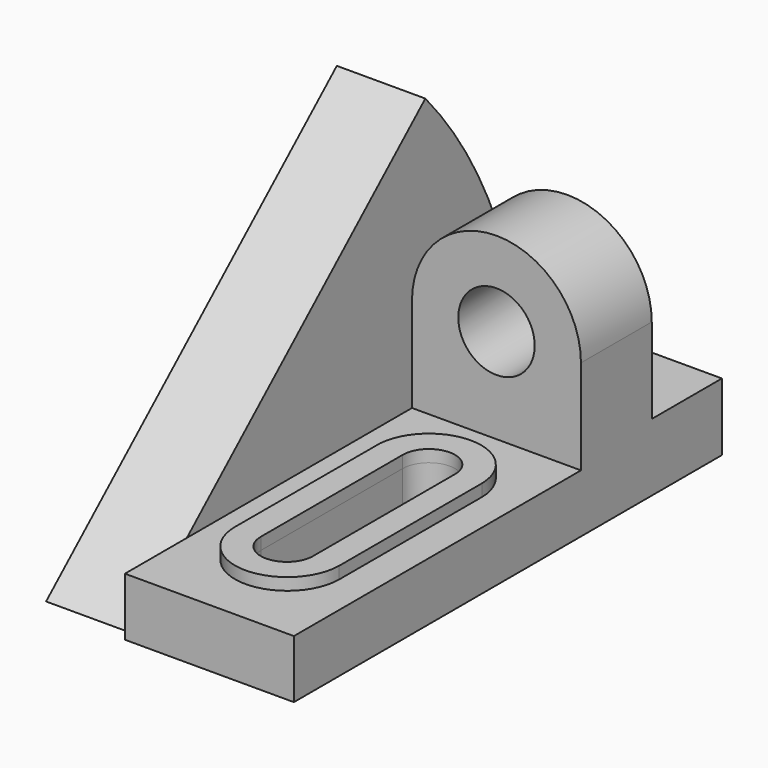
from build123d import *
from build123d import SkipClean  # not in build123d's __all__

# Parameters (mm, degrees)
F0_W          = 42
F0_H          = 16
F0_R          = 9.5
F1_DEPTH      = 133
F2_W          = 35.961864282
F2_H          = 49.2198635868
F3_DEPTH      = 23.6373633247
F3_DEPTH_BACK = 25
F4_W          = 102.4302720154
F4_H          = 59.7613004169
F5_DEPTH      = 25
F5_DEPTH_BACK = 25
F7_DEPTH      = 22
F9_DEPTH      = 25
F10_DEPTH     = 3


with BuildPart() as f1:
    # F0 (on Front) → F1 (new body)
    with BuildSketch(Plane.XZ):
        with Locations((-2.6363633247, 8)):
            Rectangle(F0_W, F0_H)
        with BuildLine():
            Line((-23.6363633247, 38), (-23.6363633247, 16))
            Line((-23.6363633247, 16), (18.3636366753, 16))
            Line((18.3636366753, 16), (18.3636366753, 38))
            ThreePointArc((18.3636366753, 38), (-2.6363633247, 59), (-23.6363633247, 38))
        make_face()
        with Locations((-2.6363633247, 38)):
            Circle(F0_R, mode=Mode.SUBTRACT)
    extrude(amount=F1_DEPTH)

    # F2 (on Right) → F3 (cut, two sides)
    with BuildSketch(Plane.YZ) as f3_sk:
        with Locations((-3.8203388158, 41.385004092)):
            Rectangle(F2_W, F2_H)
    extrude(amount=-F3_DEPTH, mode=Mode.SUBTRACT)
    extrude(f3_sk.sketch, amount=F3_DEPTH_BACK, mode=Mode.SUBTRACT)

    # F4 (on Right) → F5 (cut, two sides)
    with BuildSketch(Plane.YZ) as f5_sk:
        with Locations((-95.0164069645, 44.3436447531)):
            Rectangle(F4_W, F4_H)
    extrude(amount=-F5_DEPTH, mode=Mode.SUBTRACT)
    extrude(f5_sk.sketch, amount=F5_DEPTH_BACK, mode=Mode.SUBTRACT)

    # F6 (on face) → F7 (join)
    with BuildSketch(Plane(origin=(-23.6363633247, 0, 0), x_dir=(0, -1, 0), z_dir=(-1, 0, 0))):
        with BuildLine():
            Line((9, 0), (130, 0))
            Line((130, 0), (39.6567079743, 80.4927921367))
            ThreePointArc((39.6567079743, 80.4927921367), (16.9236135723, 43.0665860319), (9, 0))
        make_face()
    extrude(amount=F7_DEPTH)

    # F8 (on face) → F9 (cut)
    with BuildSketch(Plane.XY.offset(14.4629945447)):
        with BuildLine():
            Line((3.8636366753, -108.4778859565), (3.8636366753, -64.8012709567))
            ThreePointArc((3.8636366753, -64.8012709567), (-2.6363633247, -58.3012709567), (-9.1363633247, -64.8012709567))
            Line((-9.1363633247, -64.8012709567), (-9.1363633247, -108.9152499387))
            ThreePointArc((-9.1363633247, -108.9152499387), (-2.410200406, -115.4189274994), (3.8636366753, -108.4778859565))
        make_face()
    extrude(amount=-F9_DEPTH, mode=Mode.SUBTRACT)

    # F8 (on face) → F10 (join)
    with BuildSketch(Plane.XY.offset(14.4629945447)):
        with BuildLine():
            Line((10.3631370038, -108.9152499387), (10.3595433171, -64.4750646478))
            ThreePointArc((10.3595433171, -64.4750646478), (-2.2592864442, -51.8067408373), (-15.5914860736, -63.7220144708))
            Line((-15.5914860736, -63.7220144708), (-15.6358636533, -108.9152499387))
            ThreePointArc((-15.6358636533, -108.9152499387), (-2.6363633247, -121.8012709567), (10.3631370038, -108.9152499387))
        make_face()
        with BuildLine():
            ThreePointArc((-9.1363633247, -64.8012709567), (-2.6363633247, -58.3012709567), (3.8636366753, -64.8012709567))
            Line((3.8636366753, -64.8012709567), (3.8636366753, -108.4778859565))
            ThreePointArc((3.8636366753, -108.4778859565), (-2.410200406, -115.4189274994), (-9.1363633247, -108.9152499387))
            Line((-9.1363633247, -108.9152499387), (-9.1363633247, -64.8012709567))
        make_face(mode=Mode.SUBTRACT)
    with SkipClean():  # cleaning this boolean's faces spoils the solid; the shape is the same uncleaned
        extrude(amount=F10_DEPTH)


solid = f1.part
